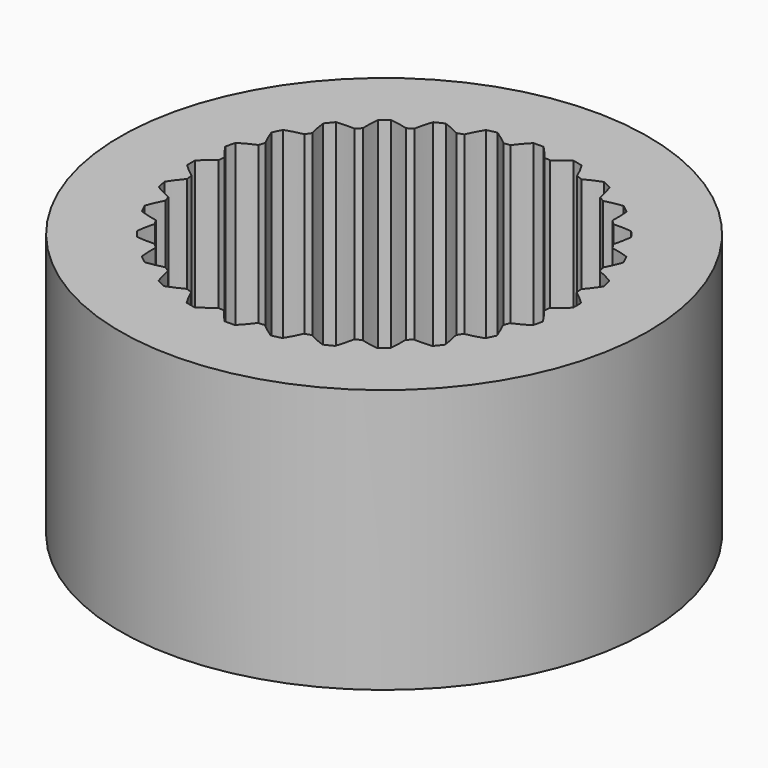
from build123d import *

# Parameters (mm, degrees)
F4_D            = 14
F6_DEPTH        = 56.501
F6_COPIES_COUNT = 28
F7_W            = 322.2772181034
F7_H            = 20
F8_DEPTH        = 25
F8_DEPTH_BACK   = 25


# Not quite as in the source:
# - a pattern or mirror of a feature is missing from the dataset's text; its kind, count and spacing are read off the source's solid


with BuildPart() as f1:
    # F0 (on Front) → F1 (revolve)
    with BuildSketch(Plane.XZ):
        with BuildLine():
            Line((27, 3.2320508076), (27, 12))
            Line((27, 12), (24, 12))
            Line((24, 12), (24, 2))
            ThreePointArc((24, 2), (23.4142135624, 0.5857864376), (22, 0))
            Line((22, 0), (14.625, 0))
            Line((14.625, 0), (13.625, -1.7320508076))
            Line((13.625, -1.7320508076), (13.625, -43.9019237886))
            Line((13.625, -43.9019237886), (15.125, -46.5))
            Line((15.125, -46.5), (15.125, -51.5203539282))
            Line((15.125, -51.5203539282), (18, -56.5))
            Line((18, -56.5), (20, -56.5))
            Line((20, -56.5), (20, -16.5))
            ThreePointArc((20, -16.5), (20.5857864376, -15.0857864376), (22, -14.5))
            Line((22, -14.5), (26, -14.5))
            ThreePointArc((26, -14.5), (27.7573593129, -10.2573593129), (32, -8.5))
            Line((32, -8.5), (62, -8.5))
            Line((62, -8.5), (62, 0))
            Line((62, 0), (28, 0))
            Line((28, 0), (28, 1.5))
            Line((28, 1.5), (27, 3.2320508076))
        make_face()
    revolve(axis=Axis((0, 0, 48.0407155993), (0, 0, 1)))

    # F4 (through all)
    with Locations(Plane.XY):
        with Locations((0, 50), (50, 0), (-50, 0), (0, -50)):
            Hole(F4_D / 2)

    # F5 (on face) → F6 (cut, through all)
    with BuildSketch(Plane.XY):
        with BuildLine():
            ThreePointArc((-1.2834802048, 13.5644131301), (0, 13.625), (1.2834802048, 13.5644131301))
            add(Edge.make_bspline(
                [(0.3838731854, 14.6199612304), (0.5234919382, 14.4822789021), (0.8167357013, 14.1694967572), (1.119440569, 13.782126507), (1.2834802048, 13.5644131301)],
                knots=[0.4618654003, 0.4618654003, 0.4618654003, 0.4618654003, 0.6403079542, 0.848481816, 0.848481816, 0.848481816, 0.848481816], degree=3))
            ThreePointArc((0.3838731854, 14.6199612304), (0, 14.625), (-0.3838731854, 14.6199612304))
            add(Edge.make_bspline(
                [(-0.3838731854, 14.6199612304), (-0.5234919382, 14.4822789021), (-0.8167357013, 14.1694967572), (-1.119440569, 13.782126507), (-1.2834802048, 13.5644131301)],
                knots=[0.4618654003, 0.4618654003, 0.4618654003, 0.4618654003, 0.6403079542, 0.848481816, 0.848481816, 0.848481816, 0.848481816], degree=3))
        make_face()
    f6 = extrude(amount=-F6_DEPTH, mode=Mode.SUBTRACT)

    # F6_copies: F6 ×28 about axis
    f6_copies_axis = Axis((0, 0, 0), (0, 0, 1))
    for i in range(1, F6_COPIES_COUNT):
        add(f6.rotate(f6_copies_axis, i * 360 / F6_COPIES_COUNT), mode=Mode.SUBTRACT)


with BuildPart() as f8:
    # F7 (on Front) → F8 (new body, two sides)
    with BuildSketch(Plane.XZ) as f8_sk:
        with Locations((-1.8415898085, -26.5)):
            Rectangle(F7_W, F7_H)
    extrude(amount=F8_DEPTH)
    extrude(f8_sk.sketch, amount=-F8_DEPTH_BACK)

    # F9: intersect F1
    add(f1.part, mode=Mode.INTERSECT)


solid = f8.part
